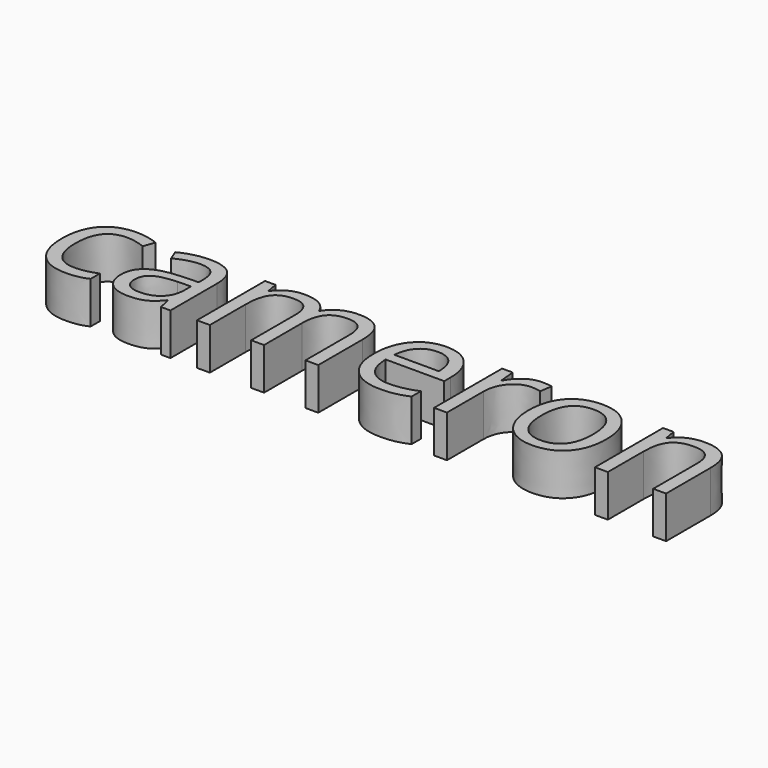
from build123d import *

# Parameters (mm, degrees)
F0_TEXT_SIZE = 96.1991233958
F1_DEPTH     = 25.4


# Not quite as in the source:
# - Text() gives the source's letters only with a copy of the font that has no kerning and outlines rounded to 1/6400 em; it was checked with that copy


with BuildPart() as f1:
    # F0 (on Top) → F1 (new body)
    with BuildSketch(Plane.XY):
        with Locations((-215.7711982727, -47.6748943329)):
            Text('cameron', F0_TEXT_SIZE, font='Open Sans', text_align=(TextAlign.LEFT, TextAlign.BOTTOM))
    extrude(amount=F1_DEPTH)


solid = f1.part
